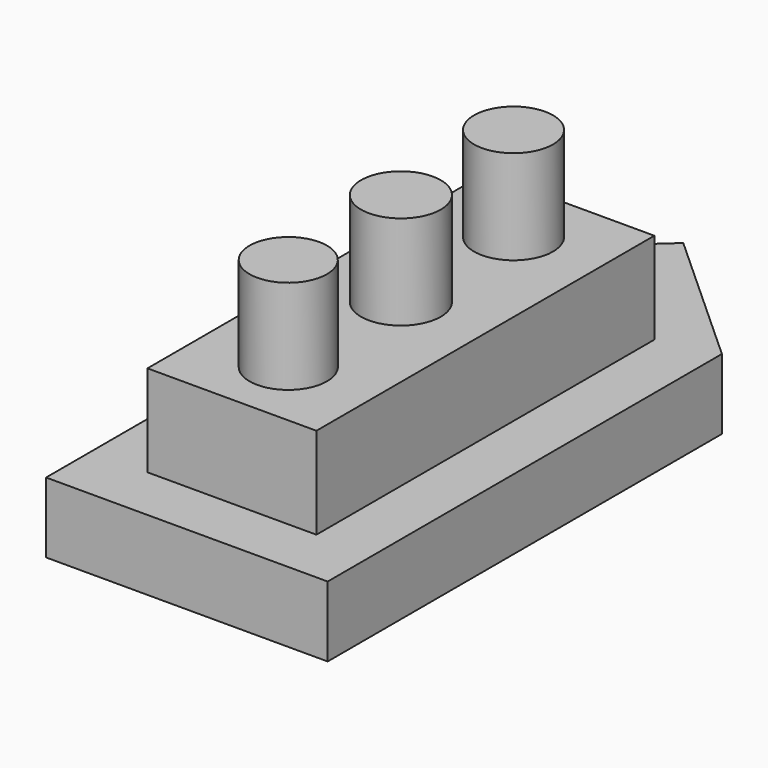
from build123d import *

# Parameters (mm, degrees)
F1_DEPTH     = 10
F2_W         = 24
F2_H         = 60
F3_DEPTH     = 13
F4_R         = 5.6085244306
F4_R_2       = 5.6654666085
F4_R_3       = 5.5
F5_DEPTH     = 13.4
F6_TEXT_SIZE = 10.2293173162
F7_DEPTH     = 5


# Not quite as in the source:
# - Text() gives the source's letters only with a copy of the font that has no kerning and outlines rounded to 1/6400 em; it was checked with that copy


with BuildPart() as f1:
    # F0 (on Top) → F1 (new body)
    with BuildSketch(Plane.XY):
        Polygon((0, 55.9230113635), (-20, 37.7846542163), (-20, -32.2153457837), (20, -32.2153457837), (20, 37.7846542163), align=None)
    extrude(amount=F1_DEPTH)

    # F2 (on face) → F3 (join)
    with BuildSketch(Plane.XY.offset(10)):
        with Locations((0, 5.7846542163)):
            Rectangle(F2_W, F2_H)
    extrude(amount=F3_DEPTH)

    # F4 (on face) → F5 (join)
    with BuildSketch(Plane.XY.offset(23)):
        with Locations((0, 25.7846542163)):
            Circle(F4_R)
        with Locations((0, 5.7846542163)):
            Circle(F4_R_2)
        with Locations((0, -14.2153457837)):
            Circle(F4_R_3)
    extrude(amount=F5_DEPTH)

    # F6 (on face) → F7 (cut)
    with BuildSketch(Plane(origin=(-12, 0, 0), x_dir=(0, -1, 0), z_dir=(-1, 0, 0))):
        with Locations((-32.4348025024, 13.4554868564)):
            Text('sabic', F6_TEXT_SIZE, font='Arimo', text_align=(TextAlign.LEFT, TextAlign.BOTTOM))
    extrude(amount=-F7_DEPTH, mode=Mode.SUBTRACT)


solid = f1.part
